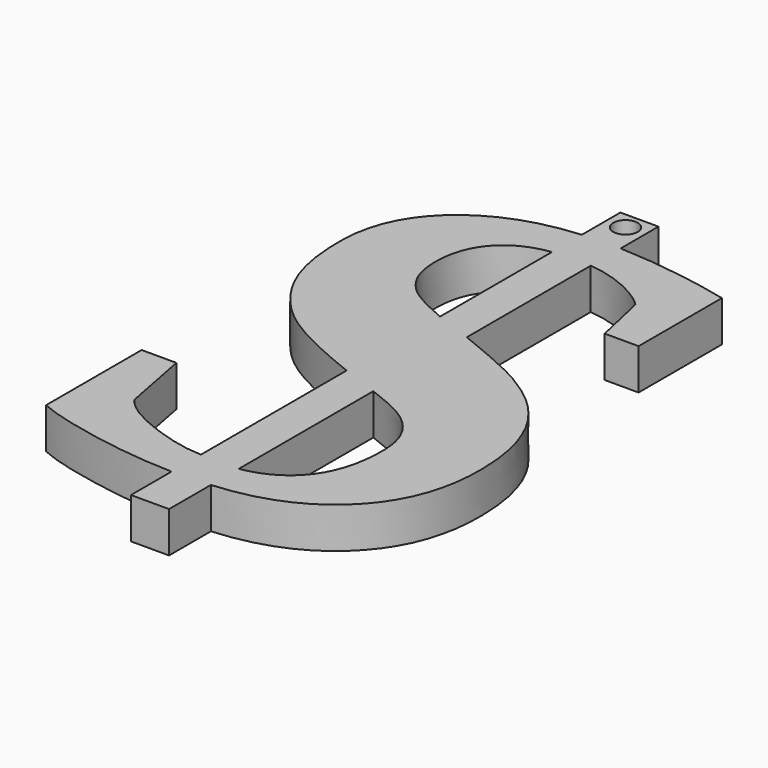
from build123d import *

# Parameters (mm, degrees)
F0_TEXT_SIZE = 47.5460661012
F1_DEPTH     = 2.54
F2_R         = 0.7648907139
F3_DEPTH     = 25.4


# Not quite as in the source:
# - Text() gives the source's letters only with a copy of the font that has no kerning and outlines rounded to 1/6400 em; it was checked with that copy


with BuildPart() as f1:
    # F0 (on Top) → F1 (new body)
    with BuildSketch(Plane.XY):
        with Locations((0, 0)):
            Text('$', F0_TEXT_SIZE, font='Tinos', font_style=FontStyle.BOLD, text_align=(TextAlign.LEFT, TextAlign.BOTTOM))
    extrude(amount=F1_DEPTH)

    # F2 (on face) → F3 (cut)
    with BuildSketch(Plane.XY.offset(2.54)):
        with Locations((11.9857546882, 33.3635656537)):
            Circle(F2_R)
    extrude(amount=-F3_DEPTH, mode=Mode.SUBTRACT)


solid = f1.part
